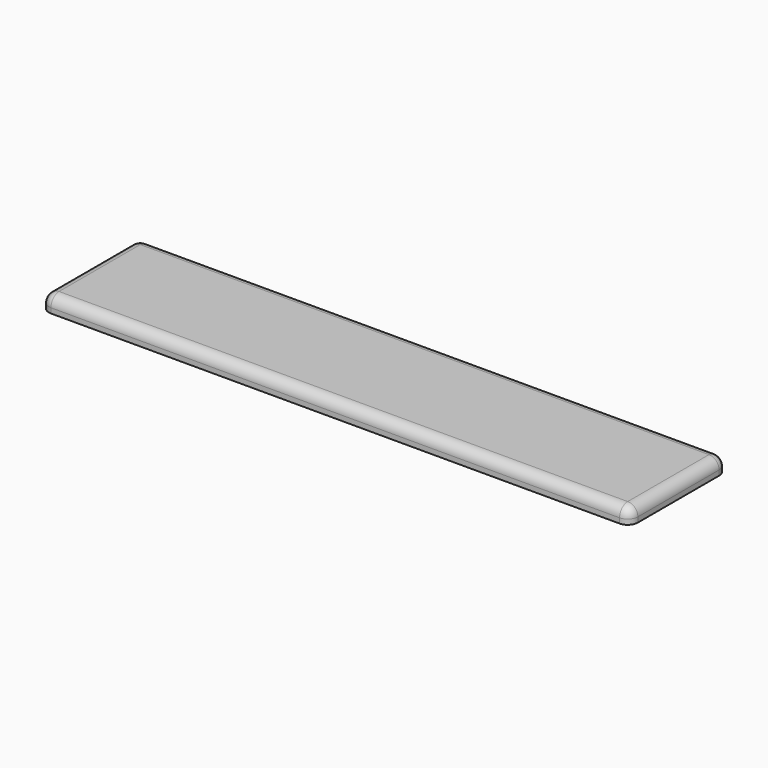
from build123d import *

# Parameters (mm, degrees)
F0_W         = 116
F0_H         = 24
F1_DEPTH     = 3
F2_R         = 2
F3_T1_DEPTH  = 6
F3_S5_W      = 2
F3_S5_H      = 2
F3_T6_DEPTH  = 2
F3_S11_W     = 2
F3_S11_H     = 2
F3_T12_DEPTH = 2
F3_S17_W     = 2
F3_S17_H     = 2
F3_T18_DEPTH = 2
F3_S23_W     = 2
F3_S23_H     = 2
F3_T24_DEPTH = 2


# Not quite as in the source:
# - a fillet or chamfer that OpenCascade refuses, or shapes differently, is made with other operations: its cross-section is extruded or revolved along the edge and cut away or added


with BuildPart() as f1:
    # F0 (on Top) → F1 (new body)
    with BuildSketch(Plane.XY):
        Rectangle(F0_W, F0_H)
    extrude(amount=F1_DEPTH)

    # F2
    f2_edges = [f1.edges().sort_by_distance(p)[0] for p in [
        (58, 0, 3),
        (0, 12, 3),
        (-58, 0, 3),
        (0, -12, 3),
    ]]
    fillet(f2_edges, radius=F2_R)

    # F3: fillet of radius 2 on 4 edges, made by hand

    # F3_s2 → F3_t1 (cut)
    with BuildSketch(Plane.XY.offset(-5)):
        with BuildLine():
            ThreePointArc((58, -10), (57.4142135624, -11.4142135624), (56, -12))
            Line((56, -12), (58, -12))
            Line((58, -12), (58, -10))
        make_face()
        with BuildLine():
            ThreePointArc((58, 10), (57.4142135624, 11.4142135624), (56, 12))
            Line((56, 12), (58, 12))
            Line((58, 12), (58, 10))
        make_face()
        with BuildLine():
            ThreePointArc((-56, -12), (-57.4142135624, -11.4142135624), (-58, -10))
            Line((-58, -10), (-58, -12))
            Line((-58, -12), (-56, -12))
        make_face()
        with BuildLine():
            ThreePointArc((-56, 12), (-57.4142135624, 11.4142135624), (-58, 10))
            Line((-58, 10), (-58, 12))
            Line((-58, 12), (-56, 12))
        make_face()
    extrude(amount=F3_T1_DEPTH, mode=Mode.SUBTRACT)


with BuildPart() as f3_tool4:
    # F3_s5 → F3_t6 (new body)
    with BuildSketch(Plane.XZ.offset(-10)):
        with Locations((-57, 2)):
            Rectangle(F3_S5_W, F3_S5_H)
    extrude(amount=-F3_T6_DEPTH)

    # F3_s7 → F3_t8 (revolve, cut)
    with BuildSketch(Plane(origin=(-56, 10, 1), x_dir=(0.7071067812, 0, -0.7071067812), z_dir=(0.7071067812, 0, 0.7071067812))):
        with BuildLine():
            ThreePointArc((0, -2), (2, 0), (0, 2))
            Line((0, 2), (0, -2))
        make_face()
    revolve(axis=Axis((-56, 10, 1), (0, 1, 0)), mode=Mode.SUBTRACT)


with BuildPart() as f1_1:
    add(f1.part)

    # F3_t3: cut F3_tool4
    add(f3_tool4.part, mode=Mode.SUBTRACT)


with BuildPart() as f3_tool10:
    # F3_s11 → F3_t12 (new body)
    with BuildSketch(Plane.XZ.offset(10)):
        with Locations((-57, 2)):
            Rectangle(F3_S11_W, F3_S11_H)
    extrude(amount=F3_T12_DEPTH)

    # F3_s13 → F3_t14 (revolve, cut)
    with BuildSketch(Plane(origin=(-56, -10, 1), x_dir=(0.7071067812, 0, -0.7071067812), z_dir=(-0.7071067812, 0, -0.7071067812))):
        with BuildLine():
            ThreePointArc((0, -2), (2, 0), (0, 2))
            Line((0, 2), (0, -2))
        make_face()
    revolve(axis=Axis((-56, -10, 1), (0, -1, 0)), mode=Mode.SUBTRACT)


with BuildPart() as f1_2:
    add(f1_1.part)

    # F3_t9: cut F3_tool10
    add(f3_tool10.part, mode=Mode.SUBTRACT)


with BuildPart() as f3_tool16:
    # F3_s17 → F3_t18 (new body)
    with BuildSketch(Plane.YZ.offset(56)):
        with Locations((11, 2)):
            Rectangle(F3_S17_W, F3_S17_H)
    extrude(amount=F3_T18_DEPTH)

    # F3_s19 → F3_t20 (revolve, cut)
    with BuildSketch(Plane(origin=(56, 10, 1), x_dir=(0, -0.7071067812, -0.7071067812), z_dir=(0, -0.7071067812, 0.7071067812))):
        with BuildLine():
            ThreePointArc((0, -2), (2, 0), (0, 2))
            Line((0, 2), (0, -2))
        make_face()
    revolve(axis=Axis((56, 10, 1), (1, 0, 0)), mode=Mode.SUBTRACT)


with BuildPart() as f1_3:
    add(f1_2.part)

    # F3_t15: cut F3_tool16
    add(f3_tool16.part, mode=Mode.SUBTRACT)


with BuildPart() as f3_tool22:
    # F3_s23 → F3_t24 (new body)
    with BuildSketch(Plane.YZ.offset(56)):
        with Locations((-11, 2)):
            Rectangle(F3_S23_W, F3_S23_H)
    extrude(amount=F3_T24_DEPTH)

    # F3_s25 → F3_t26 (revolve, cut)
    with BuildSketch(Plane(origin=(56, -10, 1), x_dir=(0, 0.7071067812, -0.7071067812), z_dir=(0, -0.7071067812, -0.7071067812))):
        with BuildLine():
            ThreePointArc((0, -2), (2, 0), (0, 2))
            Line((0, 2), (0, -2))
        make_face()
    revolve(axis=Axis((56, -10, 1), (1, 0, 0)), mode=Mode.SUBTRACT)


with BuildPart() as f1_4:
    add(f1_3.part)

    # F3_t21: cut F3_tool22
    add(f3_tool22.part, mode=Mode.SUBTRACT)


solid = f1_4.part
